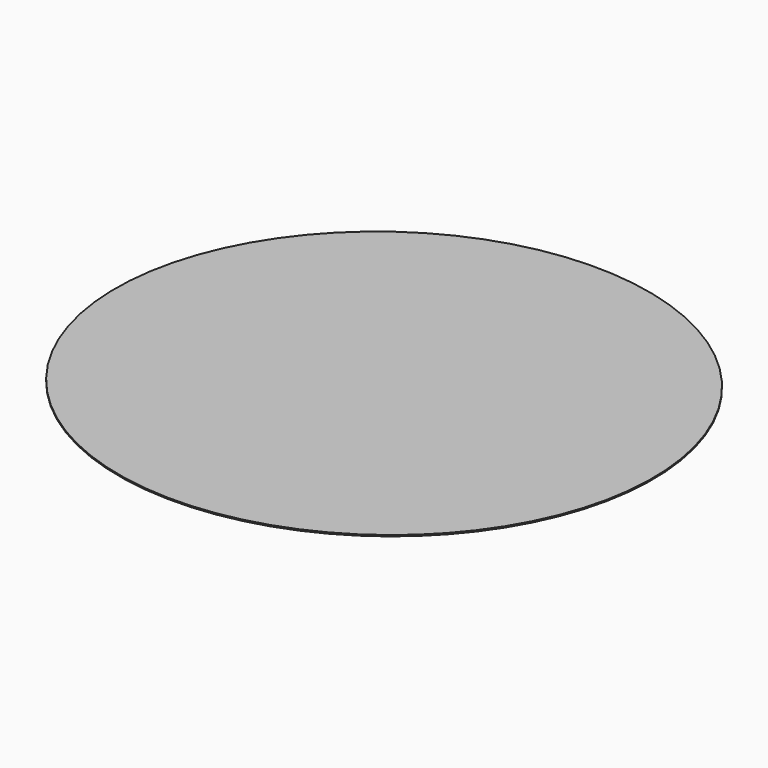
from build123d import *

# Parameters (mm, degrees)
F3_R     = 216
F6_DEPTH = 1


# Not quite as in the source:
# - the program builds the solid bodies; features that only make, move or delete a surface that nothing else refers to are left out


with BuildPart() as f6:
    # F3 (on face) → F6 (new body)
    with BuildSketch(Plane(origin=(0, 0, 0), x_dir=(1, 0, 0), z_dir=(0, 0.018515344, 0.9998285763))):
        with Locations((0, 216)):
            Circle(F3_R)
    extrude(amount=-F6_DEPTH)


solid = f6.part
